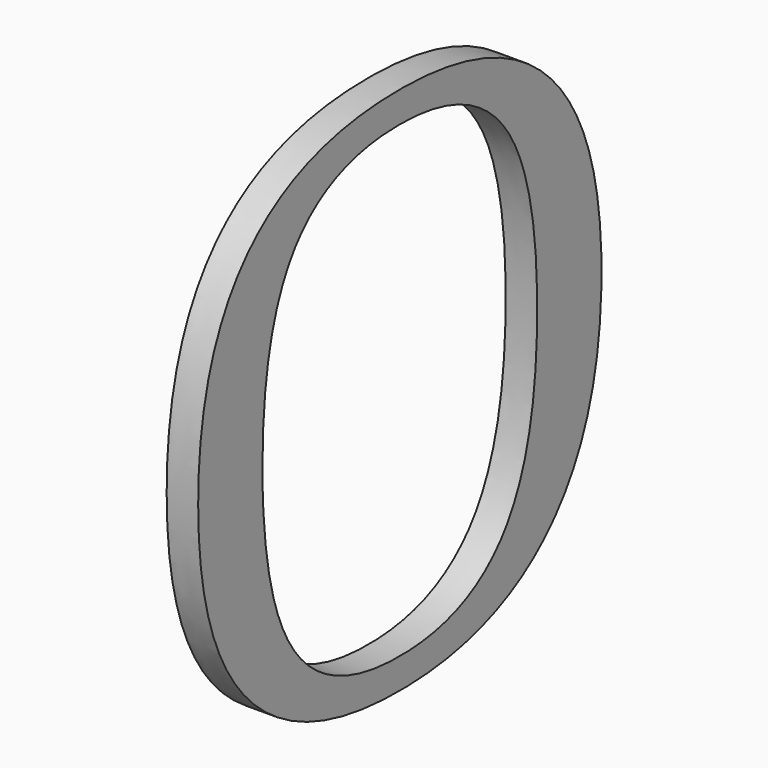
from build123d import *

# Parameters (mm, degrees)
F0_TEXT_SIZE = 635
F1_DEPTH     = 25.4


# Not quite as in the source:
# - Text() gives the source's letters only with a copy of the font that has no kerning and outlines rounded to 1/6400 em; it was checked with that copy


with BuildPart() as f1:
    # F0 (on Right) → F1 (new body)
    with BuildSketch(Plane.YZ):
        with Locations((-432.49453125, 0)):
            Text('O', F0_TEXT_SIZE, font='Tinos', text_align=(TextAlign.LEFT, TextAlign.BOTTOM))
    extrude(amount=F1_DEPTH)


solid = f1.part
